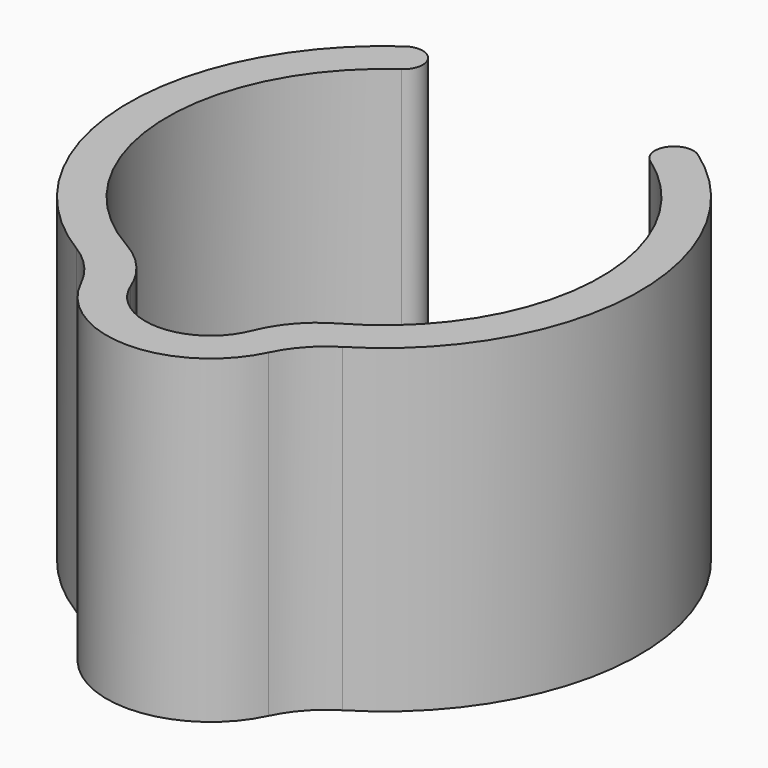
from build123d import *

# Parameters (mm, degrees)
F1_DEPTH = 7.874
F2_R     = 5.08


# Not quite as in the source:
# - a feature names something its author has since deleted; it is built from what else it names


with BuildPart() as f1:
    # F0 (on Top) → F1 (new body, symmetric)
    with BuildSketch(Plane.XY):
        with BuildLine():
            ThreePointArc((-3.175, -10.1845765253), (-10.541007581, -1.6411530025), (-6.1209836066, 8.7372640848))
            ThreePointArc((-6.1209836066, 8.7372640848), (-5.8873871353, 10.063893343), (-7.2140163934, 10.2974898143))
            ThreePointArc((-7.2140163934, 10.2974898143), (-12.5113475889, -1.2435877575), (-5.0458178338, -11.5160779516))
            ThreePointArc((-5.0458178338, -11.5160779516), (0, -15.7845920127), (5.0458178338, -11.5160779516))
            ThreePointArc((5.0458178338, -11.5160779516), (12.5113475889, -1.2435877575), (7.2140163934, 10.2974898143))
            ThreePointArc((7.2140163934, 10.2974898143), (5.8873871353, 10.063893343), (6.1209836066, 8.7372640848))
            ThreePointArc((6.1209836066, 8.7372640848), (10.541007581, -1.6411530025), (3.175, -10.1845765253))
            ThreePointArc((3.175, -10.1845765253), (0, -13.8795920127), (-3.175, -10.1845765253))
        make_face()
    extrude(amount=F1_DEPTH, both=True)

    # F2
    f2_edges = [f1.edges().sort_by_distance(p)[0] for p in [
        (-5.045818, -11.516078, 0),
        (-3.175, -10.184577, 0),
        (3.175, -10.184577, 0),
        (5.045818, -11.516078, 0),
    ]]
    fillet(f2_edges, radius=F2_R)


solid = f1.part
